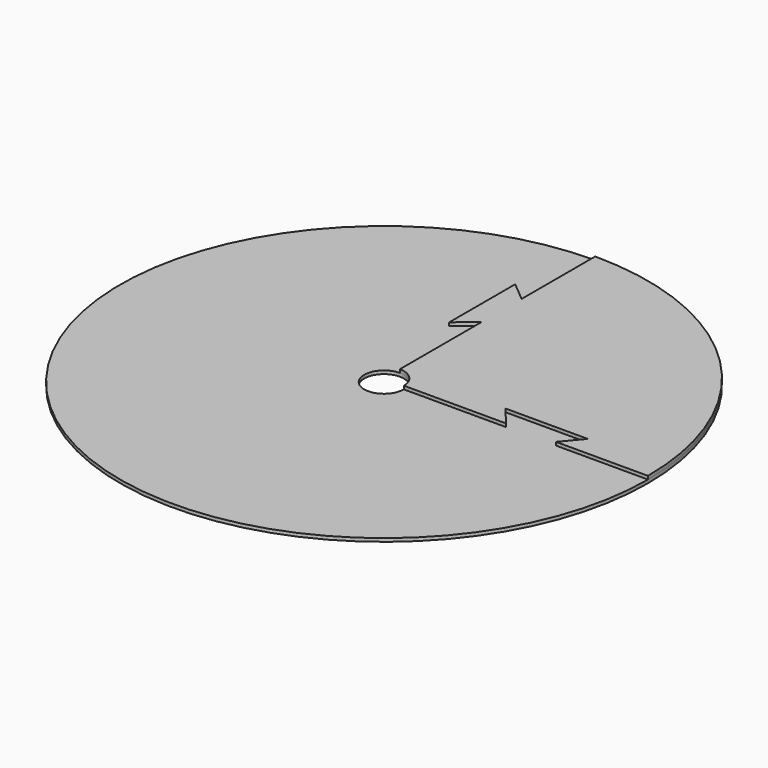
from build123d import *
from build123d import SkipClean  # not in build123d's __all__

# Parameters (mm, degrees)
F0_R     = 80
F0_R_2   = 6
F1_DEPTH = 1
F3_DEPTH = 1


with BuildPart() as f1:
    # F0 (on Top) → F1 (new body)
    with BuildSketch(Plane.XY):
        Circle(F0_R)
        Circle(F0_R_2, mode=Mode.SUBTRACT)
    extrude(amount=F1_DEPTH)

    # F2 (on face) → F3 (join)
    with BuildSketch(Plane.XY.offset(1)):
        with BuildLine():
            ThreePointArc((80, 0), (56.5685424949, 56.5685424949), (0, 80))
            Line((0, 80), (0, 52.1204726901))
            Line((0, 52.1204726901), (-5.8869810823, 57.0602363451))
            Line((-5.8869810823, 57.0602363451), (-5.8869810823, 32.0602363451))
            Line((-5.8869810823, 32.0602363451), (0, 37))
            Line((0, 37), (0, 6))
            ThreePointArc((0, 6), (4.2426406871, 4.2426406871), (6, 0))
            Line((6, 0), (37, 0))
            Line((37, 0), (32.0602363451, 5.8869810823))
            Line((32.0602363451, 5.8869810823), (57.0602363451, 5.8869810823))
            Line((57.0602363451, 5.8869810823), (52.1204726901, 0))
            Line((52.1204726901, 0), (80, 0))
        make_face()
    with SkipClean():  # cleaning this boolean's faces spoils the solid; the shape is the same uncleaned
        extrude(amount=F3_DEPTH)


solid = f1.part
